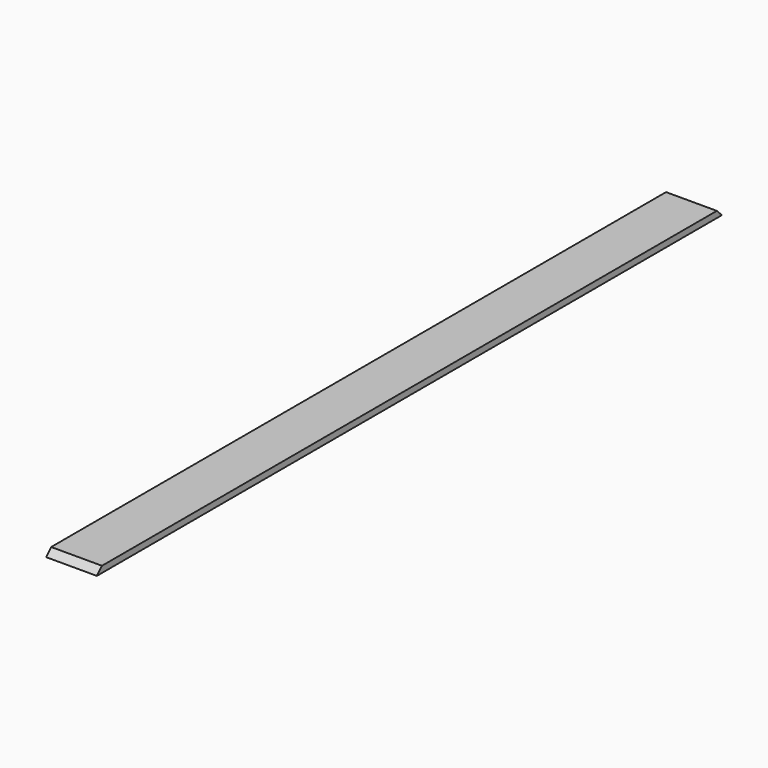
from build123d import *

# Parameters (mm, degrees)
F0_W     = 390.652
F0_H     = 3.175
F1_DEPTH = 25.4
F2_SIZE  = 3.17499
F3_SIZE  = 3.17499


# Not quite as in the source:
# - a fillet or chamfer is up to 0.001 mm smaller than in the source, because OpenCascade refuses the exact size


with BuildPart() as f1:
    # F0 (on Right) → F1 (new body)
    with BuildSketch(Plane.YZ):
        with Locations((-195.326, 1.5875)):
            Rectangle(F0_W, F0_H)
    extrude(amount=F1_DEPTH)

    # F2 (size 3.175 in the source; OpenCascade refuses exactly that, so slightly less here)
    f2_edges = [f1.edges().sort_by_distance(p)[0] for p in [
        (12.7, 0, 3.175),
    ]]
    chamfer(f2_edges, length=F2_SIZE)

    # F3 (size 3.175 in the source; OpenCascade refuses exactly that, so slightly less here)
    f3_edges = [f1.edges().sort_by_distance(p)[0] for p in [
        (12.7, -390.652, 3.175),
    ]]
    chamfer(f3_edges, length=F3_SIZE)


solid = f1.part
